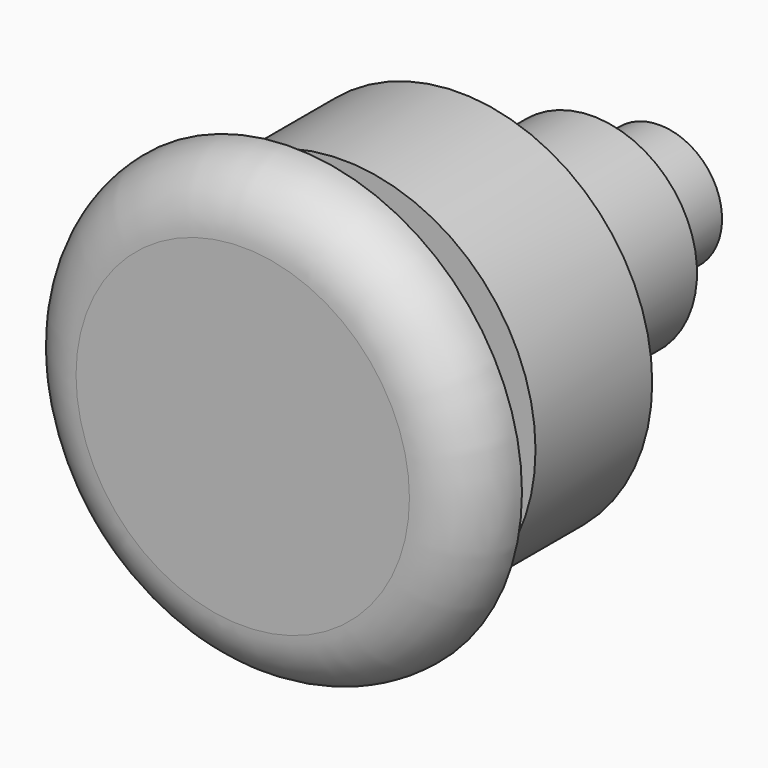
from build123d import *

# Parameters (mm, degrees)
F0_R     = 15.875
F1_DEPTH = 9.525
F2_R     = 29.36875
F3_DEPTH = 22.225
F4_R     = 15.875
F5_DEPTH = 25.4
F6_R     = 9.525
F7_DEPTH = 12.7
F8_R     = 34.925
F9_DEPTH = 9.525
F10_R    = 9.52499


# Not quite as in the source:
# - a fillet or chamfer is up to 0.001 mm smaller than in the source, because OpenCascade refuses the exact size


with BuildPart() as f1:
    # F0 (on Front) → F1 (new body)
    with BuildSketch(Plane.XZ):
        Circle(F0_R)
    extrude(amount=-F1_DEPTH)

    # F2 (on face) → F3 (join)
    with BuildSketch(Plane(origin=(0, 9.525, 0), x_dir=(-1, 0, 0), z_dir=(0, 1, 0))):
        Circle(F2_R)
    extrude(amount=F3_DEPTH)

    # F4 (on face) → F5 (join)
    with BuildSketch(Plane(origin=(0, 31.75, 0), x_dir=(-1, 0, 0), z_dir=(0, 1, 0))):
        Circle(F4_R)
    extrude(amount=F5_DEPTH)

    # F6 (on face) → F7 (join)
    with BuildSketch(Plane(origin=(0, 57.15, 0), x_dir=(-1, 0, 0), z_dir=(0, 1, 0))):
        Circle(F6_R)
    extrude(amount=F7_DEPTH)

    # F8 (on face) → F9 (join)
    with BuildSketch(Plane.XZ):
        Circle(F8_R)
    extrude(amount=F9_DEPTH)

    # F10 (radius 9.525 in the source; OpenCascade refuses exactly that, so slightly less here)
    f10_edges = [f1.edges().sort_by_distance(p)[0] for p in [
        (-34.925, -9.525, 0),
    ]]
    fillet(f10_edges, radius=F10_R)


solid = f1.part
